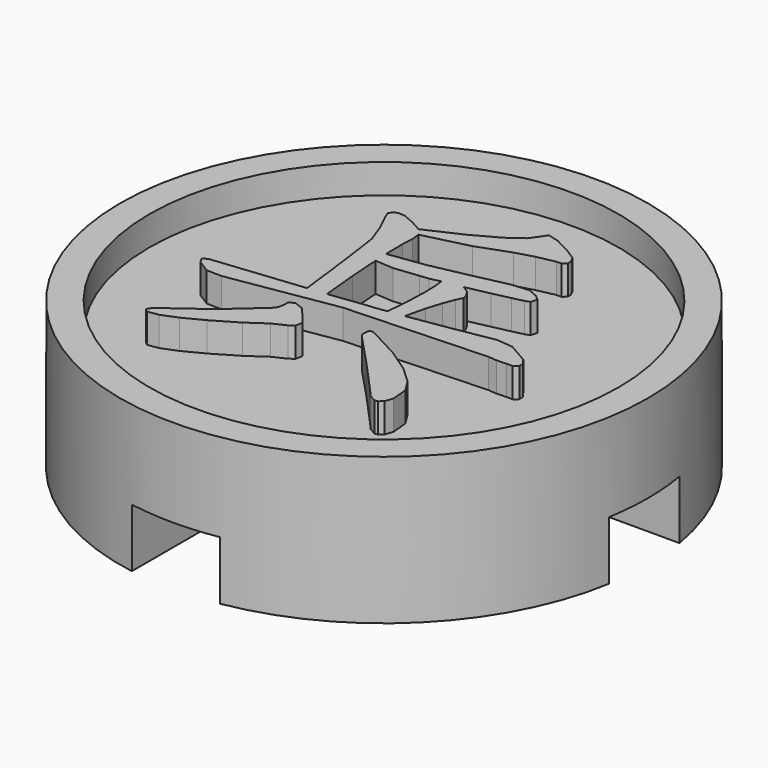
from build123d import *

# Parameters (mm, degrees)
F0_R     = 9
F1_DEPTH = 4
F3_W     = 3
F3_H     = 3
F4_DEPTH = 2
F2_R     = 9
F2_R_2   = 8
F5_DEPTH = 1
F7_DEPTH = 1


# Not quite as in the source:
# - a feature names something its author has since deleted; it is built from what else it names


with BuildPart() as f1:
    # F0 (on Top) → F1 (new body)
    with BuildSketch(Plane.XY):
        with Locations((-31.3306450844, 19.7580661625)):
            Circle(F0_R)
    extrude(amount=F1_DEPTH)

    # F3 (on face) → F4 (cut)
    with BuildSketch(Plane(origin=(0, 0, 0), x_dir=(1, 0, 0), z_dir=(0, 0, -1))):
        with BuildLine():
            ThreePointArc((-32.8306450844, -28.6321858371), (-32.0832814269, -28.7265408676), (-31.3306450844, -28.7580661625))
            ThreePointArc((-31.3306450844, -28.7580661625), (-30.5780087419, -28.7265408676), (-29.8306450844, -28.6321858371))
            Line((-29.8306450844, -28.6321858371), (-29.8306450844, -21.2580661625))
            Line((-29.8306450844, -21.2580661625), (-32.8306450844, -21.2580661625))
            Line((-32.8306450844, -21.2580661625), (-32.8306450844, -28.6321858371))
        make_face()
        with BuildLine():
            ThreePointArc((-40.204764759, -18.2580661625), (-40.2991197895, -19.0054298199), (-40.3306450844, -19.7580661625))
            ThreePointArc((-40.3306450844, -19.7580661625), (-40.2991197895, -20.510702505), (-40.204764759, -21.2580661625))
            Line((-40.204764759, -21.2580661625), (-32.8306450844, -21.2580661625))
            Line((-32.8306450844, -21.2580661625), (-32.8306450844, -18.2580661625))
            Line((-32.8306450844, -18.2580661625), (-40.204764759, -18.2580661625))
        make_face()
        with Locations((-31.3306450844, -19.7580661625)):
            Rectangle(F3_W, F3_H)
        with BuildLine():
            Line((-29.8306450844, -18.2580661625), (-29.8306450844, -21.2580661625))
            Line((-29.8306450844, -21.2580661625), (-22.4565254097, -21.2580661625))
            ThreePointArc((-22.4565254097, -21.2580661625), (-22.3621703793, -20.510702505), (-22.3306450844, -19.7580661625))
            ThreePointArc((-22.3306450844, -19.7580661625), (-22.3621703793, -19.0054298199), (-22.4565254097, -18.2580661625))
            Line((-22.4565254097, -18.2580661625), (-29.8306450844, -18.2580661625))
        make_face()
        with BuildLine():
            Line((-32.8306450844, -10.8839464878), (-32.8306450844, -18.2580661625))
            Line((-32.8306450844, -18.2580661625), (-29.8306450844, -18.2580661625))
            Line((-29.8306450844, -18.2580661625), (-29.8306450844, -10.8839464878))
            ThreePointArc((-29.8306450844, -10.8839464878), (-30.5780087419, -10.7895914574), (-31.3306450844, -10.7580661625))
            ThreePointArc((-31.3306450844, -10.7580661625), (-32.0832814269, -10.7895914574), (-32.8306450844, -10.8839464878))
        make_face()
    extrude(amount=-F4_DEPTH, mode=Mode.SUBTRACT)

    # F2 (on face) → F5 (join)
    with BuildSketch(Plane.XY.offset(4)):
        with Locations((-31.3306450844, 19.7580661625)):
            Circle(F2_R)
        with Locations((-31.3306450844, 19.7580661625)):
            Circle(F2_R_2, mode=Mode.SUBTRACT)
    extrude(amount=F5_DEPTH)

    # F6 (on face) → F7 (join)
    with BuildSketch(Plane.XY.offset(4)):
        Polygon((-33.5311048114, 20.2471387647), (-33.3884463109, 19.0475286451), (-36.4782309787, 18.7233090579), (-36.6460120564, 18.6325285146), (-36.5527999544, 18.4574668773), (-36.1151093936, 18.1818667), (-35.5996001325, 18.1688972107), (-31.940004334, 18.7654525459), (-27.1472810179, 18.9729526111), (-26.8433067742, 18.9470136325), (-26.5182754911, 18.9599831218), (-26.3042936222, 18.9607948177), (-26.1681286891, 19.0734676237), (-26.1713637091, 19.2331364476), (-26.3172925208, 19.4268553276), (-27.0038225852, 19.8199867228), (-27.5623046758, 19.8775230241), (-28.8218450116, 19.6546301455), (-30.3473039921, 19.4138858383), (-30.18602354, 20.0915166568), (-30.0238608098, 20.6159310458), (-29.880402377, 20.9895817386), (-29.7734114426, 21.2100336476), (-29.8042323605, 21.3373169803), (-29.9225752742, 21.5375353096), (-30.1624961218, 21.6996392213), (-29.3754451629, 21.8673897134), (-28.780495574, 21.9970846065), (-28.3971162937, 22.088665082), (-28.2398943213, 22.1405430392), (-28.1782524855, 22.3642887867), (-28.3590018762, 22.5125703402), (-28.6807981392, 22.649558733), (-29.2765711877, 22.5985042354), (-30.3861830508, 22.3512898882), (-31.7138705535, 22.078960022), (-32.9734520623, 21.9006221917), (-32.9856098557, 22.6074446543), (-32.960482573, 23.0029993736), (-32.999385159, 23.3045032384), (-31.4617801489, 23.6870590591), (-30.3732429707, 24.0826137783), (-29.7652944833, 24.2577165886), (-29.1574048143, 24.3841764617), (-28.9807139033, 24.3874114817), (-28.8559009495, 24.4975786176), (-28.8615475299, 24.6426839697), (-28.956421844, 24.8250802796), (-29.338154205, 25.0698242479), (-29.860992257, 25.3405660134), (-30.2597819962, 25.4540269879), (-30.3861830508, 25.2530440175), (-30.6026352986, 24.9539517131), (-31.1318963358, 24.5729839931), (-31.9878296934, 24.1077292973), (-33.1874221675, 23.554129146), (-33.564325526, 23.7632878942), (-33.9655444712, 23.9335087652), (-34.1811556138, 23.9440372849), (-34.3189557025, 23.9075697866), (-34.4056660024, 23.7616409749), (-34.3319251918, 23.5671280446), (-34.0466140726, 22.9738253749), (-33.8164159306, 22.3512898882), (-33.7499509741, 21.8957990709), (-33.6534885593, 21.1954466483), align=None)
        Polygon((-31.2348405543, 19.2906962764), (-31.5663359955, 19.2615222777), (-32.7594584296, 19.1123702098), (-32.8794306171, 20.3597939252), (-32.9475130837, 21.4240155165), (-32.3266362799, 21.3794898775), (-31.491783489, 21.4726584538), (-31.189438519, 21.502655912), (-30.8368507473, 21.5861782468), (-30.8019713497, 21.3049079617), (-30.78820781, 20.8445116777), (-30.8093236679, 20.1960725034), (-30.875765097, 19.3490442736), align=None, mode=Mode.SUBTRACT)
        Polygon((-33.2968599535, 17.7190588557), (-33.4014158002, 17.5788295611), (-34.506992711, 16.59725979), (-35.8881580354, 15.5816534911), (-35.9829911765, 15.4219770208), (-35.8622190568, 15.3287649188), (-35.4999026976, 15.3879328466), (-34.9779175146, 15.5938112845), (-34.3051745173, 15.940721302), (-33.4889613235, 16.4213746931), (-32.8721312356, 16.846909225), (-32.4449733118, 17.0503566924), (-32.2763817145, 17.1662645184), (-32.2309973247, 17.4037443963), (-32.4352388425, 17.6704218003), (-32.7724279189, 18.0554362362), (-33.0869306823, 18.1818667), (-33.2644274074, 18.0910861567), (-33.2619982015, 17.9289881268), align=None)
        Polygon((-30.5726378404, 17.8665698862), (-30.4478248866, 17.7182471597), (-29.4719075777, 16.6815585296), (-28.392293173, 15.4941144379), (-28.1758409251, 15.2452784634), (-27.9383904565, 15.1147812853), (-27.8313407034, 15.1342343429), (-27.7016458104, 15.2412252774), (-27.6108887945, 15.5224832106), (-27.6627667517, 16.0841914985), (-27.9318615979, 16.5113435404), (-28.4684631895, 17.0130716164), (-29.2895112678, 17.5723359936), (-30.4121220294, 18.1688972107), (-30.5321118624, 18.1867427574), (-30.5742259411, 18.0684057255), align=None)
    extrude(amount=F7_DEPTH)


solid = f1.part
